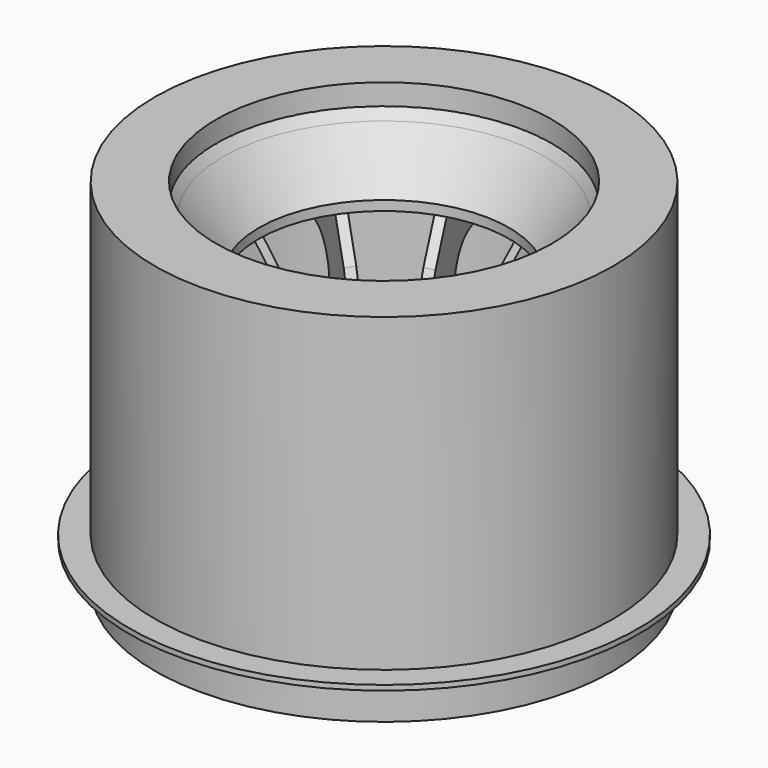
from build123d import *

# Parameters (mm, degrees)
F0_R      = 22.5
F0_R_2    = 21.75
F1_DEPTH  = 35
F0_R_3    = 8
F0_R_4    = 5
F2_DEPTH  = 4
F3_R      = 8
F3_R_2    = 5
F3_R_3    = 3
F4_DEPTH  = 2
F5_R      = 8
F5_R_2    = 5
F6_DEPTH  = 4
F7_R      = 21.75
F7_R_2    = 16.5
F8_DEPTH  = 3
F12_DEPTH = 35
F9_W      = 2.5
F9_H      = 0.5


with BuildPart() as f1:
    # F0 (on Top) → F1 (new body)
    with BuildSketch(Plane.XY):
        Circle(F0_R)
        Circle(F0_R_2, mode=Mode.SUBTRACT)
    extrude(amount=F1_DEPTH)

    # F7 (on face) → F8 (join)
    with BuildSketch(Plane.XY.offset(35)):
        Circle(F7_R)
        Circle(F7_R_2, mode=Mode.SUBTRACT)
    extrude(amount=-F8_DEPTH)

    # F9 (on Front) → F14 (revolve)
    with BuildSketch(Plane.XZ):
        with Locations((-23.75, 4.25)):
            Rectangle(F9_W, F9_H)
    revolve(axis=Axis((0, 0, 16), (0, 0, 1)))


with BuildPart() as f2:
    # F0 (on Top) → F2 (new body)
    with BuildSketch(Plane.XY):
        Circle(F0_R_3)
        Circle(F0_R_4, mode=Mode.SUBTRACT)
    extrude(amount=F2_DEPTH)

    # F3 (on face) → F4 (join)
    with BuildSketch(Plane.XY.offset(4)):
        Circle(F3_R)
        Circle(F3_R_2, mode=Mode.SUBTRACT)
        Circle(F3_R_2)
        Circle(F3_R_3, mode=Mode.SUBTRACT)
    extrude(amount=F4_DEPTH)

    # F5 (on face) → F6 (join)
    with BuildSketch(Plane.XY.offset(6)):
        Circle(F5_R)
        Circle(F5_R_2, mode=Mode.SUBTRACT)
    extrude(amount=F6_DEPTH)


with BuildPart() as f10:
    # F9 (on Front) → F10 (revolve)
    with BuildSketch(Plane.XZ):
        with BuildLine():
            Line((-8, 0.4701588427), (-8, 2))
            Line((-8, 2), (-8, 15))
            ThreePointArc((-8, 15), (-8.4761052561, 18.9383877711), (-9.8769906888, 22.6498692078))
            Line((-9.8769906888, 22.6498692078), (-12.2910935333, 26.0580144))
            Line((-12.2910935333, 26.0580144), (-16.5, 32))
            Line((-16.5, 32), (-21, 32))
            Line((-21, 32), (-21.75, 32))
            Line((-21.75, 32), (-21.75, 22.6498692078))
            Line((-21.75, 22.6498692078), (-21, 22.6498692078))
            Line((-21, 22.6498692078), (-17.6982898265, 22.6498692078))
            Line((-17.6982898265, 22.6498692078), (-17.5, 22.6498692078))
            ThreePointArc((-17.5, 22.6498692078), (-15.0251262658, 21.6247429419), (-14, 19.1498692078))
            Line((-14, 19.1498692078), (-14, 10.2254201667))
            ThreePointArc((-14, 10.2254201667), (-15.0251262658, 7.7505464325), (-17.5, 6.7254201667))
            Line((-17.5, 6.7254201667), (-21, 6.7254201667))
            Line((-21, 6.7254201667), (-21.75, 6.7254201667))
            Line((-21.75, 6.7254201667), (-21.75, 2))
            Line((-21.75, 2), (-21, 2))
            Line((-21, 2), (-9.7886873409, 2))
            ThreePointArc((-9.7886873409, 2), (-9.7496307418, 2.0004320963), (-9.7105741426, 2))
            ThreePointArc((-9.7105741426, 2), (-8.5727900166, 1.5509502259), (-8, 0.4701588427))
        make_face()
    revolve(axis=Axis((0, 0, 16), (0, 0, 1)))

    # F11 (on face) → F12 (cut)
    with BuildSketch(Plane(origin=(0, 0, 0), x_dir=(1, 0, 0), z_dir=(0, 0, -1))):
        with BuildLine():
            ThreePointArc((-7.9843597113, 0.5), (-7.6084521304, 2.472135955), (-6.7533753218, 4.2885803901))
            Line((-6.7533753218, 4.2885803901), (-17.278433248, 11.9354825832))
            Line((-17.278433248, 11.9354825832), (-17.8853621164, 12.3764422176))
            ThreePointArc((-17.8853621164, 12.3764422176), (-20.6854792294, 6.7211196277), (-21.7442521141, 0.5))
            Line((-21.7442521141, 0.5), (-20.9940467752, 0.5))
            Line((-20.9940467752, 0.5), (-7.9843597113, 0.5))
        make_face()
        with BuildLine():
            ThreePointArc((-6.1655900695, 5.0975973845), (-4.7022820183, 6.472135955), (-2.9428310982, 7.4390688347))
            Line((-2.9428310982, 7.4390688347), (-6.9630454924, 19.8120164918))
            Line((-6.9630454924, 19.8120164918), (-7.1948716914, 20.5255041679))
            ThreePointArc((-7.1948716914, 20.5255041679), (-12.7843292374, 17.5961196277), (-17.2975768641, 13.185459212))
            Line((-17.2975768641, 13.185459212), (-16.6906479957, 12.7444995776))
            Line((-16.6906479957, 12.7444995776), (-6.1655900695, 5.0975973845))
        make_face()
        with BuildLine():
            ThreePointArc((-1.9917745819, 7.7480858291), (0, 8), (1.9917745819, 7.7480858291))
            Line((1.9917745819, 7.7480858291), (6.0119889761, 20.1210334862))
            Line((6.0119889761, 20.1210334862), (6.2438151751, 20.8345211622))
            ThreePointArc((6.2438151751, 20.8345211622), (0, 21.75), (-6.2438151751, 20.8345211622))
            Line((-6.2438151751, 20.8345211622), (-6.0119889761, 20.1210334862))
            Line((-6.0119889761, 20.1210334862), (-1.9917745819, 7.7480858291))
        make_face()
        with BuildLine():
            ThreePointArc((2.9428310982, 7.4390688347), (4.7022820183, 6.472135955), (6.1655900695, 5.0975973845))
            Line((6.1655900695, 5.0975973845), (16.6906479957, 12.7444995776))
            Line((16.6906479957, 12.7444995776), (17.2975768641, 13.185459212))
            ThreePointArc((17.2975768641, 13.185459212), (12.7843292374, 17.5961196277), (7.1948716914, 20.5255041679))
            Line((7.1948716914, 20.5255041679), (6.9630454924, 19.8120164918))
            Line((6.9630454924, 19.8120164918), (2.9428310982, 7.4390688347))
        make_face()
        with BuildLine():
            ThreePointArc((6.7533753218, 4.2885803901), (7.6084521304, 2.472135955), (7.9843597113, 0.5))
            Line((7.9843597113, 0.5), (20.9940467752, 0.5))
            Line((20.9940467752, 0.5), (21.7442521141, 0.5))
            ThreePointArc((21.7442521141, 0.5), (20.6854792294, 6.7211196277), (17.8853621164, 12.3764422176))
            Line((17.8853621164, 12.3764422176), (17.278433248, 11.9354825832))
            Line((17.278433248, 11.9354825832), (6.7533753218, 4.2885803901))
        make_face()
        with BuildLine():
            Line((20.9940467752, -0.5), (7.9843597113, -0.5))
            ThreePointArc((7.9843597113, -0.5), (7.6084521304, -2.472135955), (6.7533753218, -4.2885803901))
            Line((6.7533753218, -4.2885803901), (17.278433248, -11.9354825832))
            Line((17.278433248, -11.9354825832), (17.8853621164, -12.3764422176))
            ThreePointArc((17.8853621164, -12.3764422176), (20.6854792294, -6.7211196277), (21.7442521141, -0.5))
            Line((21.7442521141, -0.5), (20.9940467752, -0.5))
        make_face()
        with BuildLine():
            Line((16.6906479957, -12.7444995776), (6.1655900695, -5.0975973845))
            ThreePointArc((6.1655900695, -5.0975973845), (4.7022820183, -6.472135955), (2.9428310982, -7.4390688347))
            Line((2.9428310982, -7.4390688347), (6.9630454924, -19.8120164918))
            Line((6.9630454924, -19.8120164918), (7.1948716914, -20.5255041679))
            ThreePointArc((7.1948716914, -20.5255041679), (12.7843292374, -17.5961196277), (17.2975768641, -13.185459212))
            Line((17.2975768641, -13.185459212), (16.6906479957, -12.7444995776))
        make_face()
        with BuildLine():
            Line((6.0119889761, -20.1210334862), (1.9917745819, -7.7480858291))
            ThreePointArc((1.9917745819, -7.7480858291), (0, -8), (-1.9917745819, -7.7480858291))
            Line((-1.9917745819, -7.7480858291), (-6.0119889761, -20.1210334862))
            Line((-6.0119889761, -20.1210334862), (-6.2438151751, -20.8345211622))
            ThreePointArc((-6.2438151751, -20.8345211622), (0, -21.75), (6.2438151751, -20.8345211622))
            Line((6.2438151751, -20.8345211622), (6.0119889761, -20.1210334862))
        make_face()
        with BuildLine():
            Line((-6.9630454924, -19.8120164918), (-2.9428310982, -7.4390688347))
            ThreePointArc((-2.9428310982, -7.4390688347), (-4.7022820183, -6.472135955), (-6.1655900695, -5.0975973845))
            Line((-6.1655900695, -5.0975973845), (-16.6906479957, -12.7444995776))
            Line((-16.6906479957, -12.7444995776), (-17.2975768641, -13.185459212))
            ThreePointArc((-17.2975768641, -13.185459212), (-12.7843292374, -17.5961196277), (-7.1948716914, -20.5255041679))
            Line((-7.1948716914, -20.5255041679), (-6.9630454924, -19.8120164918))
        make_face()
        with BuildLine():
            Line((-17.278433248, -11.9354825832), (-6.7533753218, -4.2885803901))
            ThreePointArc((-6.7533753218, -4.2885803901), (-7.6084521304, -2.472135955), (-7.9843597113, -0.5))
            Line((-7.9843597113, -0.5), (-20.9940467752, -0.5))
            Line((-20.9940467752, -0.5), (-21.7442521141, -0.5))
            ThreePointArc((-21.7442521141, -0.5), (-20.6854792294, -6.7211196277), (-17.8853621164, -12.3764422176))
            Line((-17.8853621164, -12.3764422176), (-17.278433248, -11.9354825832))
        make_face()
    extrude(amount=-F12_DEPTH, mode=Mode.SUBTRACT)


with BuildPart() as f13:
    # F9 (on Front) → F13 (revolve)
    with BuildSketch(Plane.XZ):
        Polygon((-16.5, 32), (-12.2910935333, 26.0580144), (-12.2910935333, 27.0085262903), (-15.8267207444, 32), (-16.4925991583, 32.9400636432), align=None)
    revolve(axis=Axis((0, 0, 16), (0, 0, 1)))


solid = Compound([f1.part, f2.part, f10.part, f13.part])
